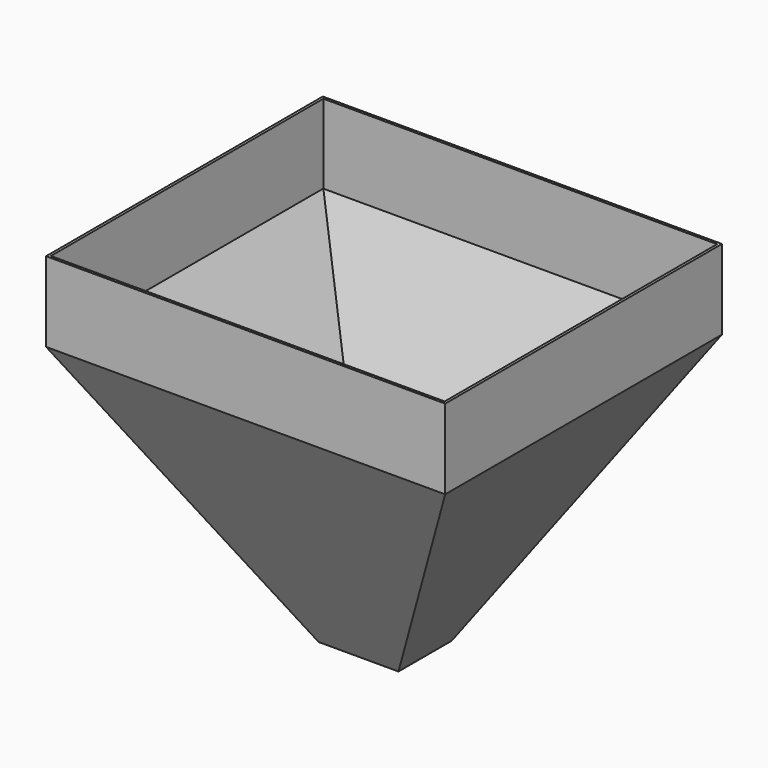
from build123d import *

# Parameters (mm, degrees)
F0_W     = 1500
F0_H     = 1300
F1_DEPTH = 300
F4_W     = 1500
F4_H     = 1300
F3_W     = 300
F3_H     = 250
F6_T     = -10


with BuildPart() as f1:
    # F0 (on Top) → F1 (new body)
    with BuildSketch(Plane.XY):
        with Locations((2.8627328575, -28.2487548455)):
            Rectangle(F0_W, F0_H)
    extrude(amount=-F1_DEPTH)

    # F4 (on face) → F5 section 0
    with BuildSketch(Plane(origin=(0, 0, -300), x_dir=(1, 0, 0), z_dir=(0, 0, -1))):
        with Locations((2.8627328575, 28.2487548455)):
            Rectangle(F4_W, F4_H)
    # F3 (on offset) → F5 section 1
    with BuildSketch(Plane.XY.offset(-1300)):
        with Locations((-0.7022507489, -18.3413977529)):
            Rectangle(F3_W, F3_H)
    loft()

    # F6
    f6_openings = [f1.faces().sort_by_distance(p)[0] for p in [
        (2.862733, -28.248755, 0),
        (-0.702251, -18.341398, -1300),
    ]]
    offset(amount=F6_T, openings=f6_openings)


solid = f1.part
